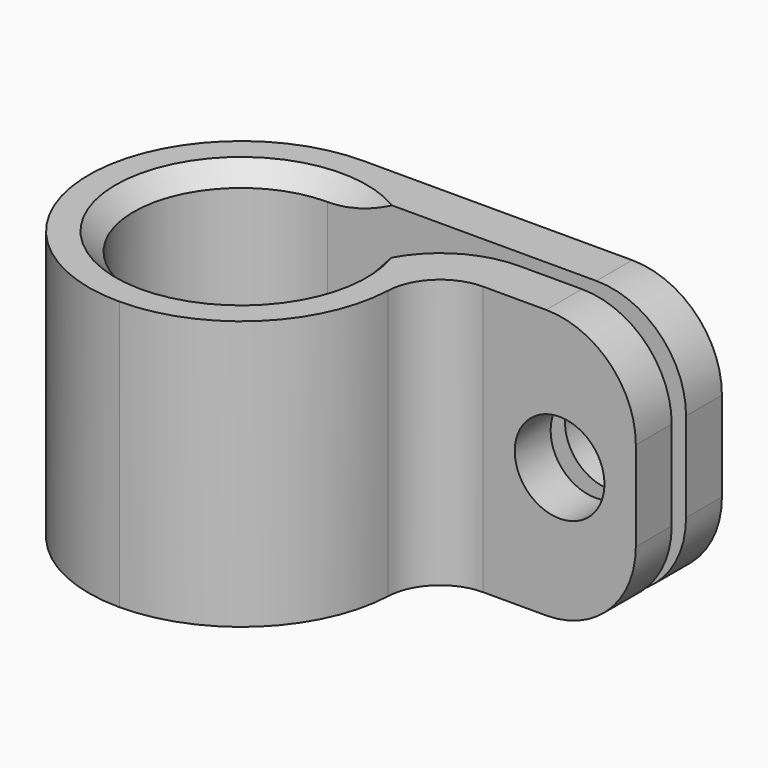
from build123d import *

# Parameters (mm, degrees)
F0_R          = 6
F1_DEPTH      = 7.5
F2_SIZE       = 1
F3_SIZE       = 1
F5_DEPTH      = 49
F5_DEPTH_BACK = 15.001
F6_R          = 3
F7_W          = 20
F7_H          = 1
F8_DEPTH      = 15.001
F9_T1_DEPTH   = 53.8625025136
F10_R         = 5
F12_D         = 5


# Not quite as in the source:
# - a fillet or chamfer that OpenCascade refuses, or shapes differently, is made with other operations: its cross-section is extruded or revolved along the edge and cut away or added
# - an extrude ends at something that could not be found from the text; its depth is read off the source's solid


with BuildPart() as f1:
    # F0 (on Top) → F1 (new body, symmetric)
    with BuildSketch(Plane.XY):
        with BuildLine():
            Line((20, 8.5), (0, 8.5))
            ThreePointArc((0, 8.5), (-8.5, 0), (0, -8.5))
            Line((0, -8.5), (20, -8.5))
            Line((20, -8.5), (20, 8.5))
        make_face()
        Circle(F0_R, mode=Mode.SUBTRACT)
    extrude(amount=F1_DEPTH, both=True)

    # F2
    f2_edges = [f1.edges().sort_by_distance(p)[0] for p in [
        (-6, 0, 7.5),
    ]]
    chamfer(f2_edges, length=F2_SIZE)

    # F3
    f3_edges = [f1.edges().sort_by_distance(p)[0] for p in [
        (-6, 0, -7.5),
    ]]
    chamfer(f3_edges, length=F3_SIZE)

    # F4 (on face) → F5 (cut, two sides)
    with BuildSketch(Plane.XY.offset(7.5)) as f5_sk:
        with BuildLine():
            ThreePointArc((8.1240384046, 2.5), (6.8373971656, -5.0497524692), (0, -8.5))
            Line((0, -8.5), (20, -8.5))
            Line((20, -8.5), (20, 2.5))
            Line((20, 2.5), (8.1240384046, 2.5))
        make_face()
    extrude(amount=F5_DEPTH, mode=Mode.SUBTRACT)
    extrude(f5_sk.sketch, amount=-F5_DEPTH_BACK, mode=Mode.SUBTRACT)

    # F6
    f6_edges = [f1.edges().sort_by_distance(p)[0] for p in [
        (8.124038, 2.5, 0),
    ]]
    fillet(f6_edges, radius=F6_R)

    # F7 (on face) → F8 (cut, through all)
    with BuildSketch(Plane.XY.offset(7.5)):
        with Locations((10, 5.5)):
            Rectangle(F7_W, F7_H)
    extrude(amount=-F8_DEPTH, mode=Mode.SUBTRACT)

    # F9: fillet of radius 5.5 on 1 edges, made by hand

    # F9_s2 → F9_t1 (cut)
    with BuildSketch(Plane.XY.offset(-26.9312512568)):
        with BuildLine():
            ThreePointArc((11.4891252931, 5), (7.6855228816, 3.4727331518), (5.9943262399, -0.2608695652))
            ThreePointArc((5.9943262399, -0.2608695652), (5.3472085631, 2.7216466675), (3.3166247904, 5))
            Line((3.3166247904, 5), (11.4891252931, 5))
        make_face()
    extrude(amount=F9_T1_DEPTH, mode=Mode.SUBTRACT)

    # F10
    f10_edges = [f1.edges().sort_by_distance(p)[0] for p in [
        (20, 7.25, -7.5),
        (20, 3.75, 7.5),
        (20, 7.25, 7.5),
        (20, 3.75, -7.5),
    ]]
    fillet(f10_edges, radius=F10_R)

    # F12 (through all)
    with Locations(Plane.XZ.offset(-2.5)):
        with Locations((15.75, 0)):
            Hole(F12_D / 2)


solid = f1.part
